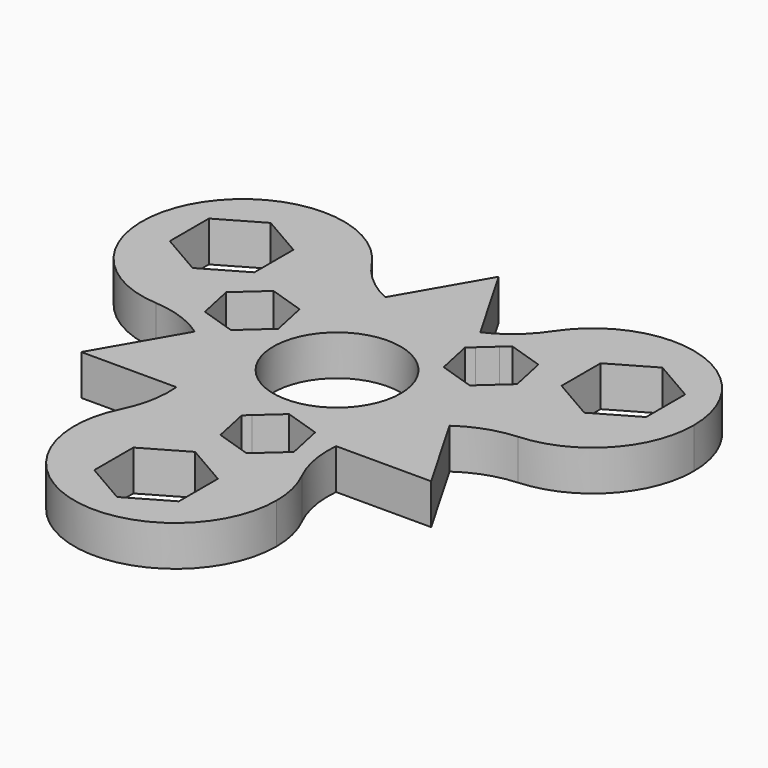
from build123d import *

# Parameters (mm, degrees)
F0_R     = 9.45
F1_DEPTH = 6


with BuildPart() as f1:
    # F0 (on Top) → F1 (new body)
    with BuildSketch(Plane.XY):
        Polygon((11.8595659331, -15), (25.9807621135, -15), (18.9201640233, -2.7706853759), (13.302852552, 6.9587834943), (9.2066626406, 8.2897162761), (8.0631483411, 13.6695280801), (8.9614312964, 14.478345686), (7.0605980902, 17.7706853759), (0, 30), (-7.0605980902, 17.7706853759), (-12.6779095615, 8.0412165057), (-11.7824362055, 3.8283455928), (-15.8697327457, 0.1481272578), (-17.0193308171, 0.521654314), (-18.9201640233, -2.7706853759), (-25.9807621135, -15), (-11.8595659331, -15), (-0.6249429905, -15), (2.5757735649, -12.1180618689), (7.8065844046, -13.8176553379), (8.0578995207, -15), align=None)
        Circle(F0_R, mode=Mode.SUBTRACT)
        with BuildLine():
            ThreePointArc((13.4207676072, -23.3005226447), (12.0614730092, -19.25910479), (11.8595659331, -15))
            Line((11.8595659331, -15), (8.0578995207, -15))
            Line((8.0578995207, -15), (8.6399217922, -17.7381995032))
            ThreePointArc((8.6399217922, -17.7381995032), (11.3755599368, -20.2226467731), (13.4207676072, -23.3005226447))
        make_face()
        with BuildLine():
            Line((13.302852552, 6.9587834943), (18.9201640233, -2.7706853759))
            ThreePointArc((18.9201640233, -2.7706853759), (22.7096105069, -0.815989638), (26.8892283353, 0.0275356362))
            ThreePointArc((26.8892283353, 0.0275356362), (19.1613457519, 1.6397769298), (13.3222745374, 6.9524729087))
            Line((13.3222745374, 6.9524729087), (13.302852552, 6.9587834943))
        make_face()
        with BuildLine():
            ThreePointArc((15, -30), (14.5998546929, -26.5584534078), (13.4207676072, -23.3005226447))
            ThreePointArc((13.4207676072, -23.3005226447), (11.3755599368, -20.2226467731), (8.6399217922, -17.7381995032))
            Line((8.6399217922, -17.7381995032), (8.9500987041, -19.1974671419))
            Line((8.9500987041, -19.1974671419), (4.8628021639, -22.8776854769))
            Line((4.8628021639, -22.8776854769), (-0.3680086757, -21.1780920079))
            Line((-0.3680086757, -21.1780920079), (-1.5115229752, -15.7982802038))
            Line((-1.5115229752, -15.7982802038), (-0.6401191106, -15.0136646399))
            ThreePointArc((-0.6401191106, -15.0136646399), (-8.1605843982, -17.4141006567), (-13.4207676072, -23.3005226447))
            ThreePointArc((-13.4207676072, -23.3005226447), (-3.4415465922, -44.5998546929), (15, -30))
        make_face()
        Polygon((6.2786841774, -37.2124443067), (0, -40.8374443067), (-6.2786841774, -37.2124443067), (-6.2786841774, -29.9624443067), (0, -26.3374443067), (6.2786841774, -29.9624443067), align=None, mode=Mode.SUBTRACT)
        with BuildLine():
            ThreePointArc((13.3222745374, 6.9524729087), (19.1613457519, 1.6397769298), (26.8892283353, 0.0275356362))
            ThreePointArc((26.8892283353, 0.0275356362), (36.903833873, 4.7196058764), (40.9807621135, 15))
            ThreePointArc((40.9807621135, 15), (30.3002226828, 29.3646183517), (13.4684607282, 23.2729870084))
            ThreePointArc((13.4684607282, 23.2729870084), (11.8255458689, 19.9628472741), (11.041770491, 16.3514915103))
            Line((11.041770491, 16.3514915103), (12.1504448812, 17.3497464151))
            Line((12.1504448812, 17.3497464151), (17.3812557208, 15.650152946))
            Line((17.3812557208, 15.650152946), (18.5247700203, 10.270341142))
            Line((18.5247700203, 10.270341142), (14.4374734802, 6.590122807))
            Line((14.4374734802, 6.590122807), (13.3222745374, 6.9524729087))
        make_face()
        Polygon((29.0875800178, 24.0437221533), (35.3662641952, 20.4187221533), (35.3662641952, 13.1687221533), (29.0875800178, 9.5437221533), (22.8088958404, 13.1687221533), (22.8088958404, 20.4187221533), align=None, mode=Mode.SUBTRACT)
        with BuildLine():
            Line((-0.6401191106, -15.0136646399), (-0.6249429905, -15))
            Line((-0.6249429905, -15), (-11.8595659331, -15))
            ThreePointArc((-11.8595659331, -15), (-12.0614730092, -19.25910479), (-13.4207676072, -23.3005226447))
            ThreePointArc((-13.4207676072, -23.3005226447), (-8.1605843982, -17.4141006567), (-0.6401191106, -15.0136646399))
        make_face()
        with BuildLine():
            Line((7.0605980902, 17.7706853759), (8.9614312964, 14.478345686))
            Line((8.9614312964, 14.478345686), (11.041770491, 16.3514915103))
            ThreePointArc((11.041770491, 16.3514915103), (11.8255458689, 19.9628472741), (13.4684607282, 23.2729870084))
            ThreePointArc((13.4684607282, 23.2729870084), (10.6481374977, 20.0750944281), (7.0605980902, 17.7706853759))
        make_face()
        with BuildLine():
            ThreePointArc((-26.8892283353, 0.0275356362), (-22.7096105069, -0.815989638), (-18.9201640233, -2.7706853759))
            Line((-18.9201640233, -2.7706853759), (-17.0193308171, 0.521654314))
            Line((-17.0193308171, 0.521654314), (-19.6816922832, 1.3867079928))
            ThreePointArc((-19.6816922832, 1.3867079928), (-23.2011058057, 0.259799499), (-26.8892283353, 0.0275356362))
        make_face()
        with BuildLine():
            Line((-12.6779095615, 8.0412165057), (-7.0605980902, 17.7706853759))
            ThreePointArc((-7.0605980902, 17.7706853759), (-10.6481374977, 20.0750944281), (-13.4684607282, 23.2729870084))
            ThreePointArc((-13.4684607282, 23.2729870084), (-11.6161437618, 19.3194605693), (-10.9807621135, 15))
            ThreePointArc((-10.9807621135, 15), (-11.4123184715, 11.4278228138), (-12.6821554268, 8.0611917312))
            Line((-12.6821554268, 8.0611917312), (-12.6779095615, 8.0412165057))
        make_face()
        with BuildLine():
            ThreePointArc((-13.4684607282, 23.2729870084), (-38.9711431703, 22.5), (-26.8892283353, 0.0275356362))
            ThreePointArc((-26.8892283353, 0.0275356362), (-23.2011058057, 0.259799499), (-19.6816922832, 1.3867079928))
            Line((-19.6816922832, 1.3867079928), (-21.1005435853, 1.8477207269))
            Line((-21.1005435853, 1.8477207269), (-22.2440578848, 7.2275325309))
            Line((-22.2440578848, 7.2275325309), (-18.1567613447, 10.9077508659))
            Line((-18.1567613447, 10.9077508659), (-12.925950505, 9.2081573968))
            Line((-12.925950505, 9.2081573968), (-12.6821554268, 8.0611917312))
            ThreePointArc((-12.6821554268, 8.0611917312), (-11.4123184715, 11.4278228138), (-10.9807621135, 15))
            ThreePointArc((-10.9807621135, 15), (-11.6161437618, 19.3194605693), (-13.4684607282, 23.2729870084))
        make_face()
        Polygon((-35.3662641952, 13.1687221533), (-35.3662641952, 20.4187221533), (-29.0875800178, 24.0437221533), (-22.8088958404, 20.4187221533), (-22.8088958404, 13.1687221533), (-29.0875800178, 9.5437221533), align=None, mode=Mode.SUBTRACT)
    extrude(amount=F1_DEPTH)


solid = f1.part
